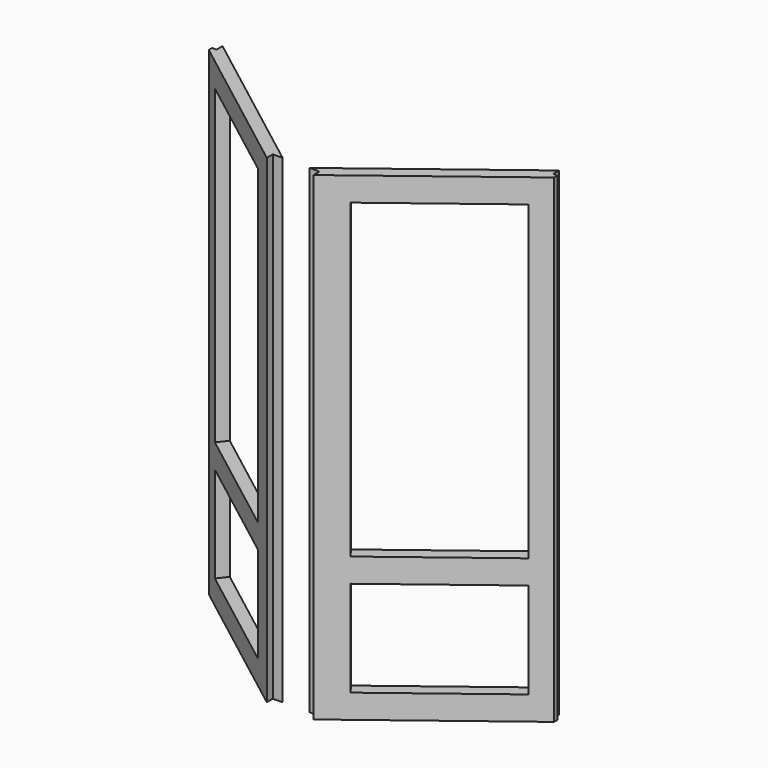
from build123d import *

# Parameters (mm, degrees)
F1_DEPTH      = 1000
F1_DEPTH_BACK = 1000
F3_W          = 580.6498229504
F3_H          = 1300
F3_H_2        = 400
F4_DEPTH      = 442.4345898662


with BuildPart() as f1:
    # F0 (on Top) → F1 (new body, two sides)
    with BuildSketch(Plane.XY) as f1_sk:
        Polygon((-320.3894793987, 231.25), (-320.3894793987, 213.4575700915), (302.5, -262.7182715976), (302.5, -231.25), (343.663901225, -231.25), (-281.9180493875, 246.9841357988), (-302.5, 262.7182715976), (-302.5, 231.25), align=None)
    extrude(amount=F1_DEPTH)
    extrude(f1_sk.sketch, amount=-F1_DEPTH_BACK)

    # F3 (on face) → F4 (cut, through all)
    with BuildSketch(Plane(origin=(-15.1832061928, -19.8612751279, 0), x_dir=(0.7944510051, -0.6073282477, 0), z_dir=(-0.6073282477, -0.7944510051, 0))):
        with Locations((-11.3382488489, 250)):
            Rectangle(F3_W, F3_H)
        with Locations((-11.3382488489, -700)):
            Rectangle(F3_W, F3_H_2)
    extrude(amount=-F4_DEPTH, mode=Mode.SUBTRACT)


with BuildPart() as f6_1:
    # F6: instance of F1
    add(f1.part.mirror(Plane.YZ.offset(400)))


solid = Compound([f1.part, f6_1.part])
